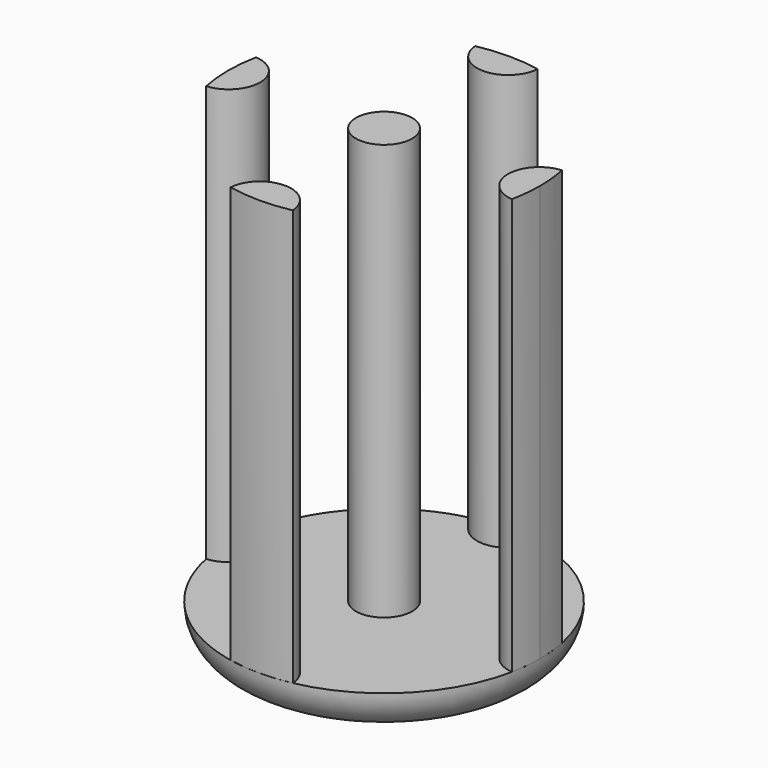
from build123d import *

# Parameters (mm, degrees)
F0_R     = 9.525
F1_DEPTH = 2.54
F2_R     = 1.7145
F3_DEPTH = 25.4
F4_R     = 2.53999


# Not quite as in the source:
# - a fillet or chamfer is up to 0.001 mm smaller than in the source, because OpenCascade refuses the exact size


with BuildPart() as f1:
    # F0 (on Top) → F1 (new body)
    with BuildSketch(Plane.XY):
        Circle(F0_R)
    extrude(amount=F1_DEPTH)

    # F2 (on face) → F3 (join)
    with BuildSketch(Plane.XY.offset(2.54)):
        with BuildLine():
            ThreePointArc((9.525, 0), (9.4767668574, 0.9573478631), (9.33255592, 1.905))
            ThreePointArc((9.33255592, 1.905), (7.5646235439, 0), (9.33255592, -1.905))
            ThreePointArc((9.33255592, -1.905), (9.4767668574, -0.9573478631), (9.525, 0))
        make_face()
        with BuildLine():
            ThreePointArc((-1.905, 9.33255592), (0, 7.5646235439), (1.905, 9.33255592))
            ThreePointArc((1.905, 9.33255592), (0, 9.525), (-1.905, 9.33255592))
        make_face()
        with BuildLine():
            ThreePointArc((-9.33255592, -1.905), (-7.5646235439, 0), (-9.33255592, 1.905))
            ThreePointArc((-9.33255592, 1.905), (-9.525, 0), (-9.33255592, -1.905))
        make_face()
        with BuildLine():
            ThreePointArc((-1.905, -9.33255592), (0, -9.525), (1.905, -9.33255592))
            ThreePointArc((1.905, -9.33255592), (0, -7.5646235439), (-1.905, -9.33255592))
        make_face()
        Circle(F2_R)
    extrude(amount=F3_DEPTH)

    # F4 (radius 2.54 in the source; OpenCascade refuses exactly that, so slightly less here)
    f4_edges = [f1.edges().sort_by_distance(p)[0] for p in [
        (-9.525, 0, 0),
    ]]
    fillet(f4_edges, radius=F4_R)


solid = f1.part
